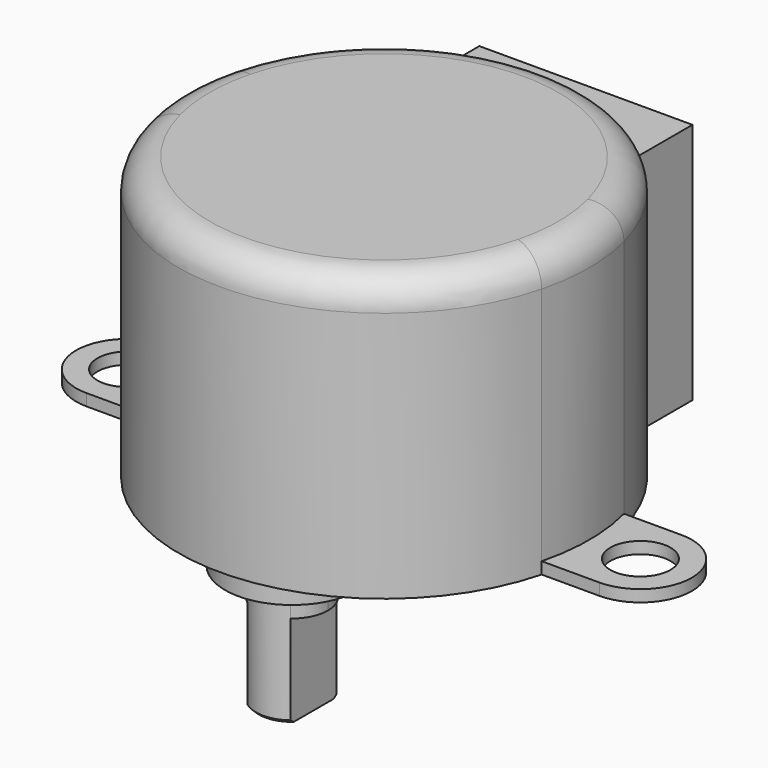
from build123d import *

# Parameters (mm, degrees)
F0_R      = 2.05
F1_DEPTH  = 0.8
F2_DEPTH  = 19.2
F3_R      = 4.55
F4_DEPTH  = 2.1
F5_DEPTH  = 4
F6_DEPTH  = 10.3
F8_W      = 14.5
F8_H      = 16.5
F12_DEPTH = 0.65
F13_R     = 2.1
F14_SIZE  = 0.2


with BuildPart() as f1:
    # F0 (on Top) → F1 (new body)
    with BuildSketch(Plane.XY):
        with BuildLine():
            ThreePointArc((-13.5296202829, -3.5), (-13.975, 0), (-13.5296202829, 3.5))
            Line((-13.5296202829, 3.5), (-17.45, 3.5))
            ThreePointArc((-17.45, 3.5), (-20.95, 0), (-17.45, -3.5))
            Line((-17.45, -3.5), (-13.5296202829, -3.5))
        make_face()
        with Locations((-17.45, 0)):
            Circle(F0_R, mode=Mode.SUBTRACT)
    extrude(amount=F1_DEPTH)



with BuildPart() as f1b:
    # F0 (on Top) → F1, piece 2 (new body)
    with BuildSketch(Plane.XY):
        with BuildLine():
            Line((17.45, 3.5), (13.5296202829, 3.5))
            ThreePointArc((13.5296202829, 3.5), (13.975, 0), (13.5296202829, -3.5))
            Line((13.5296202829, -3.5), (17.45, -3.5))
            ThreePointArc((17.45, -3.5), (20.95, 0), (17.45, 3.5))
        make_face()
        with Locations((17.45, 0)):
            Circle(F0_R, mode=Mode.SUBTRACT)
    extrude(amount=F1_DEPTH)


with BuildPart() as f1_1:
    add(f1.part)

    add(f1b.part)  # F2 merges F1b
    # F0 (on Top) → F2 (join)
    with BuildSketch(Plane.XY):
        with BuildLine():
            ThreePointArc((13.5296202829, -3.5), (13.975, 0), (13.5296202829, 3.5))
            ThreePointArc((13.5296202829, 3.5), (0, 13.975), (-13.5296202829, 3.5))
            ThreePointArc((-13.5296202829, 3.5), (-13.975, 0), (-13.5296202829, -3.5))
            ThreePointArc((-13.5296202829, -3.5), (0, -13.975), (13.5296202829, -3.5))
        make_face()
    extrude(amount=F2_DEPTH)

    # F3 (on Top) → F4 (join)
    with BuildSketch(Plane.XY):
        with Locations((0, -7.825)):
            Circle(F3_R)
        with BuildLine():
            ThreePointArc((1.475, -5.8687599841), (2.1927437151, -6.7321253503), (2.45, -7.825))
            ThreePointArc((2.45, -7.825), (2.1927437151, -8.9178746497), (1.475, -9.7812400159))
            ThreePointArc((1.475, -9.7812400159), (0, -10.275), (-1.475, -9.7812400159))
            ThreePointArc((-1.475, -9.7812400159), (-2.45, -7.825), (-1.475, -5.8687599841))
            ThreePointArc((-1.475, -5.8687599841), (0, -5.375), (1.475, -5.8687599841))
        make_face(mode=Mode.SUBTRACT)
    extrude(amount=-F4_DEPTH)

    # F3 (on Top) → F5 (join)
    with BuildSketch(Plane.XY):
        with BuildLine():
            ThreePointArc((1.475, -9.7812400159), (2.1927437151, -8.9178746497), (2.45, -7.825))
            ThreePointArc((2.45, -7.825), (2.1927437151, -6.7321253503), (1.475, -5.8687599841))
            Line((1.475, -5.8687599841), (1.475, -9.7812400159))
        make_face()
        with BuildLine():
            Line((1.475, -9.7812400159), (1.475, -5.8687599841))
            ThreePointArc((1.475, -5.8687599841), (0, -5.375), (-1.475, -5.8687599841))
            Line((-1.475, -5.8687599841), (-1.475, -9.7812400159))
            ThreePointArc((-1.475, -9.7812400159), (0, -10.275), (1.475, -9.7812400159))
        make_face()
        with BuildLine():
            Line((-1.475, -9.7812400159), (-1.475, -5.8687599841))
            ThreePointArc((-1.475, -5.8687599841), (-2.45, -7.825), (-1.475, -9.7812400159))
        make_face()
    extrude(amount=-F5_DEPTH)

    # F3 (on Top) → F6 (join)
    with BuildSketch(Plane.XY):
        with BuildLine():
            Line((1.475, -9.7812400159), (1.475, -5.8687599841))
            ThreePointArc((1.475, -5.8687599841), (0, -5.375), (-1.475, -5.8687599841))
            Line((-1.475, -5.8687599841), (-1.475, -9.7812400159))
            ThreePointArc((-1.475, -9.7812400159), (0, -10.275), (1.475, -9.7812400159))
        make_face()
    extrude(amount=-F6_DEPTH)

    # F8 (on offset) → F9 (join, up to the next surface of F1)
    with BuildSketch(Plane.XZ.offset(-17.175)):
        with Locations((0, 8.25)):
            Rectangle(F8_W, F8_H)
    extrude(until=Until.NEXT)

    # F11 (on offset) → F12 (cut, through all)
    with BuildSketch(Plane.XY.offset(17.15)):
        with BuildLine():
            Line((-8.625, 12.9959083299), (-8.625, 11.5))
            ThreePointArc((-8.625, 11.5), (-7.9506110955, 11.9761599943), (-7.25, 12.4128209928))
            Line((-7.25, 12.4128209928), (-7.25, 13.8205759578))
            ThreePointArc((-7.25, 13.8205759578), (-7.9482026537, 13.4260870893), (-8.625, 12.9959083299))
        make_face()
        with BuildLine():
            ThreePointArc((7.25, 12.4128209928), (7.9506110955, 11.9761599943), (8.625, 11.5))
            Line((8.625, 11.5), (8.625, 12.9959083299))
            ThreePointArc((8.625, 12.9959083299), (7.9482026537, 13.4260870893), (7.25, 13.8205759578))
            Line((7.25, 13.8205759578), (7.25, 12.4128209928))
        make_face()
    extrude(amount=-F12_DEPTH, mode=Mode.SUBTRACT)

    # F13
    f13_edges = [f1_1.edges().sort_by_distance(p)[0] for p in [
        (-13.52962, -3.5, 19.2),
    ]]
    fillet(f13_edges, radius=F13_R)

    # F14
    f14_edges = [f1_1.edges().sort_by_distance(p)[0] for p in [
        (0, -5.375, -10.3),
        (0, -10.275, -10.3),
    ]]
    chamfer(f14_edges, length=F14_SIZE)


solid = f1_1.part
